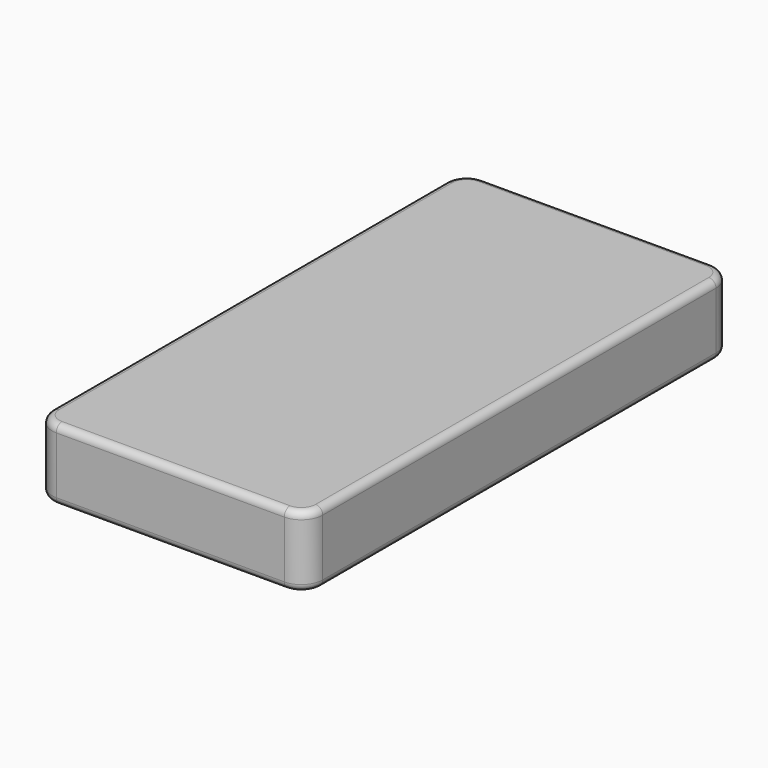
from build123d import *

# Parameters (mm, degrees)
F0_W         = 965.2
F0_H         = 1905
F1_DEPTH     = 254
F2_R         = 25.4
F3_T1_DEPTH  = 254
F3_T4_ANGLE  = 90
F3_T6_ANGLE  = 90
F3_T8_ANGLE  = 90
F3_T10_ANGLE = 90
F3_T12_ANGLE = 90
F3_T14_ANGLE = 90
F3_T16_ANGLE = 90
F3_T18_ANGLE = 90


# Not quite as in the source:
# - a fillet or chamfer that OpenCascade refuses, or shapes differently, is made with other operations: its cross-section is extruded or revolved along the edge and cut away or added


with BuildPart() as f1:
    # F0 (on Top) → F1 (new body)
    with BuildSketch(Plane.XY):
        Rectangle(F0_W, F0_H)
    extrude(amount=F1_DEPTH)

    # F2
    f2_edges = [f1.edges().sort_by_distance(p)[0] for p in [
        (0, -952.5, 254),
        (482.6, 0, 254),
        (0, 952.5, 254),
        (-482.6, 0, 254),
        (0, -952.5, 0),
        (482.6, 0, 0),
        (0, 952.5, 0),
        (-482.6, 0, 0),
    ]]
    fillet(f2_edges, radius=F2_R)

    # F3: fillet of radius 76.2 on 4 edges, made by hand

    # F3_s2 → F3_t1 (cut)
    with BuildSketch(Plane.XY):
        with BuildLine():
            ThreePointArc((406.4, -952.5), (460.281537, -930.181537), (482.6, -876.3))
            Line((482.6, -876.3), (482.6, -952.5))
            Line((482.6, -952.5), (406.4, -952.5))
        make_face()
        with BuildLine():
            ThreePointArc((406.4, 952.5), (460.281537, 930.181537), (482.6, 876.3))
            Line((482.6, 876.3), (482.6, 952.5))
            Line((482.6, 952.5), (406.4, 952.5))
        make_face()
        with BuildLine():
            ThreePointArc((-482.6, -876.3), (-460.281537, -930.181537), (-406.4, -952.5))
            Line((-406.4, -952.5), (-482.6, -952.5))
            Line((-482.6, -952.5), (-482.6, -876.3))
        make_face()
        with BuildLine():
            ThreePointArc((-482.6, 876.3), (-460.281537, 930.181537), (-406.4, 952.5))
            Line((-406.4, 952.5), (-482.6, 952.5))
            Line((-482.6, 952.5), (-482.6, 876.3))
        make_face()
    extrude(amount=F3_T1_DEPTH, mode=Mode.SUBTRACT)

    # F3_s3 → F3_t4 (revolve, cut)
    with BuildSketch(Plane.XZ.offset(-876.3)):
        with BuildLine():
            ThreePointArc((-457.2, 0), (-475.160512, 7.439488), (-482.6, 25.4))
            Line((-482.6, 25.4), (-482.6, 0))
            Line((-482.6, 0), (-457.2, 0))
        make_face()
    revolve(axis=Axis((-406.4, 876.3, 0), (0, 0, -1)), revolution_arc=F3_T4_ANGLE, mode=Mode.SUBTRACT)

    # F3_s5 → F3_t6 (revolve, cut)
    with BuildSketch(Plane.YZ.offset(-406.4)):
        with BuildLine():
            ThreePointArc((927.1, 254), (945.060512, 246.560512), (952.5, 228.6))
            Line((952.5, 228.6), (952.5, 254))
            Line((952.5, 254), (927.1, 254))
        make_face()
    revolve(axis=Axis((-406.4, 876.3, 254), (0, 0, 1)), revolution_arc=F3_T6_ANGLE, mode=Mode.SUBTRACT)

    # F3_s7 → F3_t8 (revolve, cut)
    with BuildSketch(Plane.YZ.offset(-406.4)):
        with BuildLine():
            ThreePointArc((-927.1, 0), (-945.060512, 7.439488), (-952.5, 25.4))
            Line((-952.5, 25.4), (-952.5, 0))
            Line((-952.5, 0), (-927.1, 0))
        make_face()
    revolve(axis=Axis((-406.4, -876.3, 0), (0, 0, -1)), revolution_arc=F3_T8_ANGLE, mode=Mode.SUBTRACT)

    # F3_s9 → F3_t10 (revolve, cut)
    with BuildSketch(Plane.XZ.offset(876.3)):
        with BuildLine():
            ThreePointArc((-457.2, 254), (-475.160512, 246.560512), (-482.6, 228.6))
            Line((-482.6, 228.6), (-482.6, 254))
            Line((-482.6, 254), (-457.2, 254))
        make_face()
    revolve(axis=Axis((-406.4, -876.3, 254), (0, 0, 1)), revolution_arc=F3_T10_ANGLE, mode=Mode.SUBTRACT)

    # F3_s11 → F3_t12 (revolve, cut)
    with BuildSketch(Plane.YZ.offset(406.4)):
        with BuildLine():
            ThreePointArc((927.1, 0), (945.060512, 7.439488), (952.5, 25.4))
            Line((952.5, 25.4), (952.5, 0))
            Line((952.5, 0), (927.1, 0))
        make_face()
    revolve(axis=Axis((406.4, 876.3, 0), (0, 0, -1)), revolution_arc=F3_T12_ANGLE, mode=Mode.SUBTRACT)

    # F3_s13 → F3_t14 (revolve, cut)
    with BuildSketch(Plane.XZ.offset(-876.3)):
        with BuildLine():
            ThreePointArc((457.2, 254), (475.160512, 246.560512), (482.6, 228.6))
            Line((482.6, 228.6), (482.6, 254))
            Line((482.6, 254), (457.2, 254))
        make_face()
    revolve(axis=Axis((406.4, 876.3, 254), (0, 0, 1)), revolution_arc=F3_T14_ANGLE, mode=Mode.SUBTRACT)

    # F3_s15 → F3_t16 (revolve, cut)
    with BuildSketch(Plane.XZ.offset(876.3)):
        with BuildLine():
            ThreePointArc((457.2, 0), (475.160512, 7.439488), (482.6, 25.4))
            Line((482.6, 25.4), (482.6, 0))
            Line((482.6, 0), (457.2, 0))
        make_face()
    revolve(axis=Axis((406.4, -876.3, 0), (0, 0, -1)), revolution_arc=F3_T16_ANGLE, mode=Mode.SUBTRACT)

    # F3_s17 → F3_t18 (revolve, cut)
    with BuildSketch(Plane.YZ.offset(406.4)):
        with BuildLine():
            ThreePointArc((-927.1, 254), (-945.060512, 246.560512), (-952.5, 228.6))
            Line((-952.5, 228.6), (-952.5, 254))
            Line((-952.5, 254), (-927.1, 254))
        make_face()
    revolve(axis=Axis((406.4, -876.3, 254), (0, 0, 1)), revolution_arc=F3_T18_ANGLE, mode=Mode.SUBTRACT)


solid = f1.part
